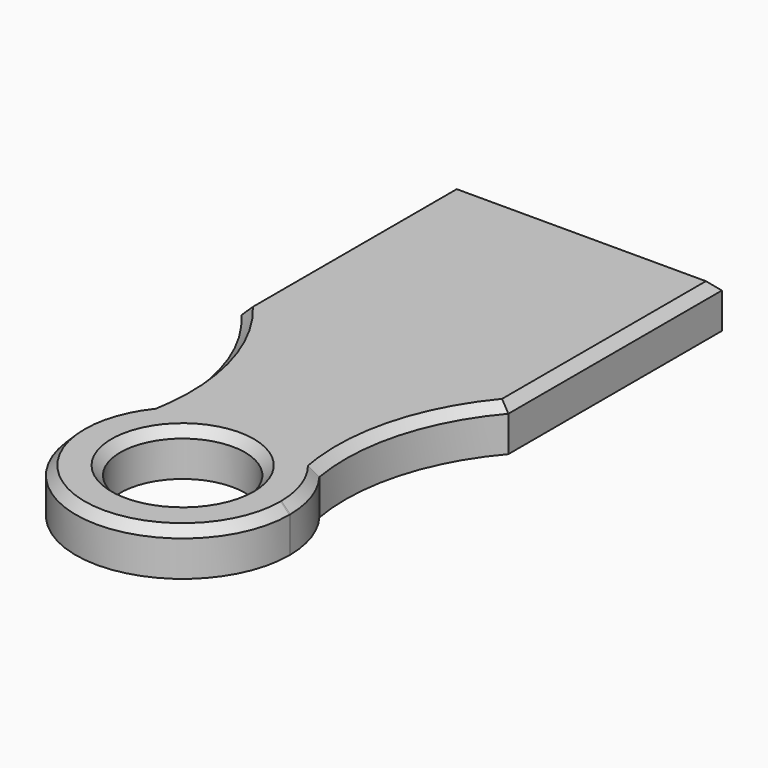
from build123d import *

# Parameters (mm, degrees)
F0_W       = 19.05
F0_H       = 19.05
F0_R       = 4.445
F1_DEPTH   = 3.175
F2_C1_SIZE = 0.635
F2_C2_SIZE = 0.635
F2_C3_SIZE = 0.635
F2_C4_SIZE = 0.635
F2_C5_SIZE = 0.635
F2_C6_SIZE = 0.635
F2_C7_SIZE = 0.6349
F3_R       = 0.635
F4_DEPTH   = 0.635


# Not quite as in the source:
# - a fillet or chamfer is up to 0.001 mm smaller than in the source, because OpenCascade refuses the exact size


with BuildPart() as f1:
    # F0 (on Top) → F1 (new body)
    with BuildSketch(Plane.XY):
        Rectangle(F0_W, F0_H)
        with BuildLine():
            Line((9.525, -9.525), (-9.525, -9.525))
            ThreePointArc((-9.525, -9.525), (-6.3836187271, -15.3786997104), (-6.0310725347, -22.012687032))
            ThreePointArc((-6.0310725347, -22.012687032), (0.0350329382, -19.0500805324), (6.0736411029, -22.0683390224))
            ThreePointArc((6.0736411029, -22.0683390224), (6.3936440411, -15.409890989), (9.525, -9.525))
        make_face()
        with BuildLine():
            ThreePointArc((6.0736411029, -22.0683390224), (0.0350329382, -19.0500805324), (-6.0310725347, -22.012687032))
            ThreePointArc((-6.0310725347, -22.012687032), (-6.6363180101, -24.4058987838), (-7.62, -26.67))
            ThreePointArc((-7.62, -26.67), (0, -34.29), (7.62, -26.67))
            ThreePointArc((7.62, -26.67), (7.619882327, -26.6276523681), (7.6195293118, -26.5853060441))
            ThreePointArc((7.6195293118, -26.5853060441), (6.6686101992, -24.3877327559), (6.0736411029, -22.0683390224))
        make_face()
        with Locations((0, -26.67)):
            Circle(F0_R, mode=Mode.SUBTRACT)
        with BuildLine():
            ThreePointArc((-7.62, -26.67), (-6.6363180101, -24.4058987838), (-6.0310725347, -22.012687032))
            ThreePointArc((-6.0310725347, -22.012687032), (-7.2118365454, -24.2095501137), (-7.62, -26.67))
        make_face()
        with BuildLine():
            ThreePointArc((7.6195293118, -26.5853060441), (7.2094713239, -24.202628275), (6.0736411029, -22.0683390224))
            ThreePointArc((6.0736411029, -22.0683390224), (6.6686101992, -24.3877327559), (7.6195293118, -26.5853060441))
        make_face()
    extrude(amount=F1_DEPTH)

    # F2: chamfer of 0.635 on 7 edges, made by hand

    # F2_c1
    f2_c1_edges = [f1.edges().sort_by_distance(p)[0] for p in [
        (0, 9.525, 3.175),
    ]]
    chamfer(f2_c1_edges, length=F2_C1_SIZE)

    # F2_c2
    f2_c2_edges = [f1.edges().sort_by_distance(p)[0] for p in [
        (-9.525, -0.3175, 3.175),
    ]]
    chamfer(f2_c2_edges, length=F2_C2_SIZE)

    # F2_c3
    f2_c3_edges = [f1.edges().sort_by_distance(p)[0] for p in [
        (-6.2554888364, -15.867774564, 3.175),
    ]]
    chamfer(f2_c3_edges, length=F2_C3_SIZE)

    # F2_c4
    f2_c4_edges = [f1.edges().sort_by_distance(p)[0] for p in [
        (6.3936440411, -15.409890989, 3.175),
    ]]
    chamfer(f2_c4_edges, length=F2_C4_SIZE)

    # F2_c5
    f2_c5_edges = [f1.edges().sort_by_distance(p)[0] for p in [
        (9.525, 0.1573240758, 3.175),
    ]]
    chamfer(f2_c5_edges, length=F2_C5_SIZE)

    # F2_c6
    f2_c6_edges = [f1.edges().sort_by_distance(p)[0] for p in [
        (-4.445, -26.67, 3.175),
    ]]
    chamfer(f2_c6_edges, length=F2_C6_SIZE)

    # F2_c7 (size 0.635 in the source; OpenCascade refuses exactly that, so slightly less here)
    f2_c7_edges = [f1.edges().sort_by_distance(p)[0] for p in [
        (-0.0350329382, -34.2899194676, 3.175),
    ]]
    chamfer(f2_c7_edges, length=F2_C7_SIZE)

    # F3 (on face) → F4 (cut)
    with BuildSketch(Plane(origin=(0, 0, 0), x_dir=(1, 0, 0), z_dir=(0, 0, -1))):
        Circle(F3_R)
    extrude(amount=-F4_DEPTH, mode=Mode.SUBTRACT)


solid = f1.part
